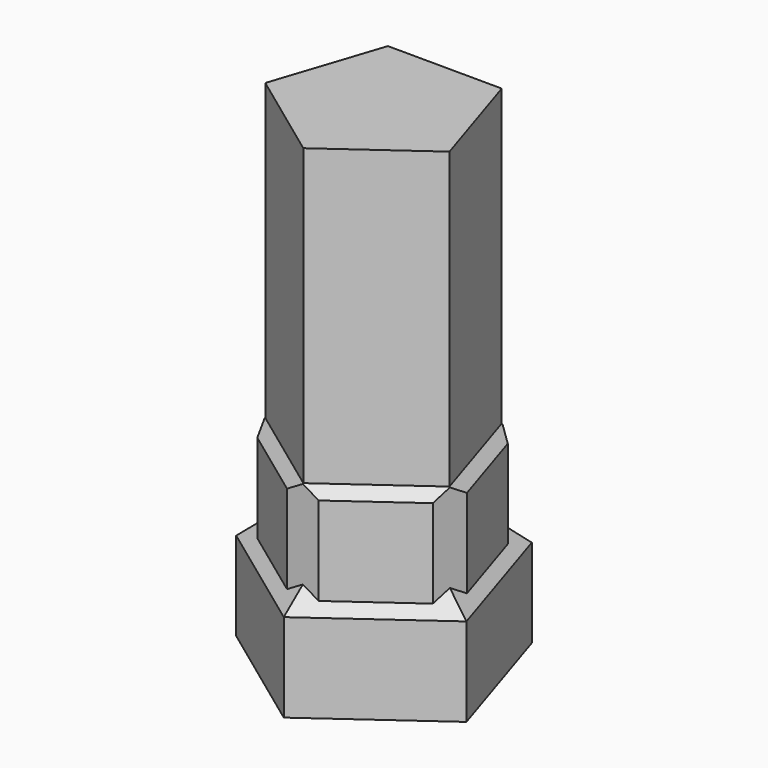
from build123d import *

# Parameters (mm, degrees)
F1_DEPTH = 12.7
F2_SIZE  = 1.27
F3_DEPTH = 12.7
F4_SIZE  = 1.27
F5_DEPTH = 38.1
F6_SIZE  = 2.54


# Not quite as in the source:
# - two fillets or chamfers of one size are made in one step
# - a feature of the source that left no trace in its solid (it failed there, or was rolled back) is left out


with BuildPart() as f1:
    # F0 (on Top) → F1 (new body)
    with BuildSketch(Plane.XY):
        Polygon((-32.2221838869, -58.9305205708), (-17.2413629738, -48.1540753293), (-22.8610431915, -30.5763632619), (-41.315017485, -30.4891850014), (-47.1005206082, -48.0130179407), align=None)
    extrude(amount=F1_DEPTH)

    # F2
    f2_edges = [f1.edges().sort_by_distance(p)[0] for p in [
        (-39.661352, -53.471769, 12.7),
        (-24.731773, -53.542298, 12.7),
        (-20.051203, -39.365219, 12.7),
        (-32.08803, -30.532774, 12.7),
        (-44.207769, -39.251101, 12.7),
    ]]
    chamfer(f2_edges, length=F2_SIZE)

    # F3 (add): a face of the model
    f3_faces = [f1.faces().sort_by_distance(p)[0] for p in [
        (-32.1480256291, -43.2326324208, 12.7),
    ]]
    extrude(f3_faces, amount=F3_DEPTH)

    # F4
    f4_edges = [f1.edges().sort_by_distance(p)[0] for p in [
        (-38.91002, -52.447856, 25.4),
        (-43.001795, -39.649255, 25.4),
        (-25.473399, -52.511331, 25.4),
        (-32.09403, -31.80276, 25.4),
        (-21.260885, -39.751961, 25.4),
    ]]
    chamfer(f4_edges, length=F4_SIZE)

    # F5 (add): a face of the model
    f5_faces = [f1.faces().sort_by_distance(p)[0] for p in [
        (-32.1480256291, -43.2326324208, 25.4),
    ]]
    extrude(f5_faces, amount=F5_DEPTH)

    # F6
    f6_edges = [f1.edges().sort_by_distance(p)[0] for p in [
        (-45.605271, -47.534979, 18.415),
        (-32.214768, -57.360732, 18.415),
        (-40.398318, -31.76353, 18.415),
        (-18.732029, -47.661931, 18.415),
        (-23.789741, -31.84199, 18.415),
    ]]
    chamfer(f6_edges, length=F6_SIZE)


solid = f1.part
